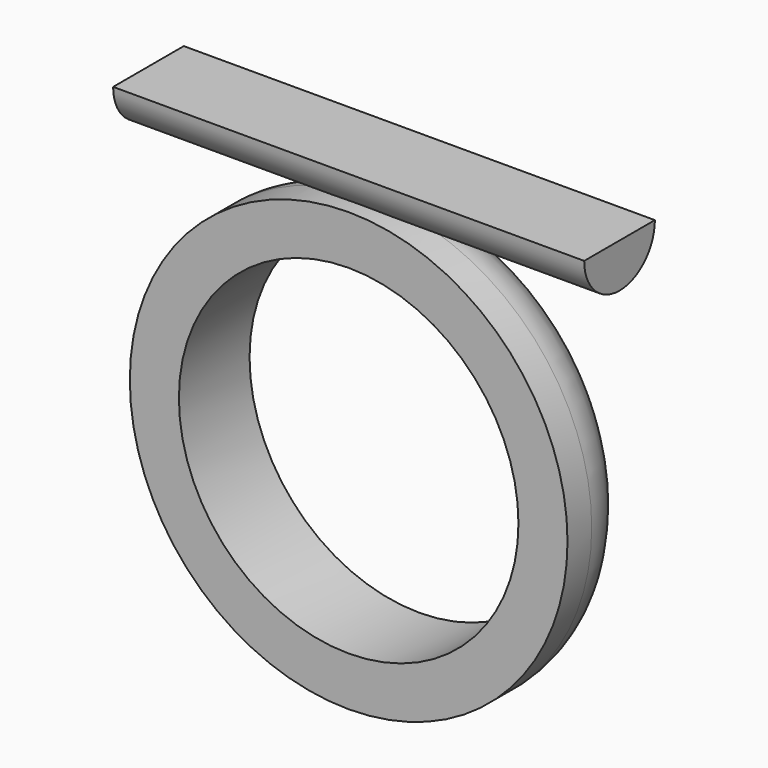
from build123d import *

# Parameters (mm, degrees)
F0_R          = 8.65
F1_DEPTH      = 2.25
F1_DEPTH_BACK = 2.25
F3_DEPTH      = 12
F3_DEPTH_BACK = 12
F4_S5_R       = 2.25
F4_T6_DEPTH   = 19


# Not quite as in the source:
# - a fillet or chamfer that OpenCascade refuses, or shapes differently, is made with other operations: its cross-section is extruded or revolved along the edge and cut away or added
# - a feature names something its author has since deleted; it is built from what else it names


with BuildPart() as f1:
    # F0 (on Front) → F1 (new body, two sides)
    with BuildSketch(Plane.XZ) as f1_sk:
        with BuildLine():
            ThreePointArc((-11.15, 0), (0, -11.15), (11.15, 0))
            ThreePointArc((11.15, 0), (7.8842406102, 7.8842406102), (0, 11.15))
            ThreePointArc((0, 11.15), (-7.8842406102, 7.8842406102), (-11.15, 0))
        make_face()
        Circle(F0_R, mode=Mode.SUBTRACT)
    extrude(amount=F1_DEPTH)
    extrude(f1_sk.sketch, amount=-F1_DEPTH_BACK)

    # F2 (on Right) → F3 (join, two sides)
    with BuildSketch(Plane.YZ) as f3_sk:
        with BuildLine():
            ThreePointArc((-2.25, 12.8644379824), (0, 10.6144379824), (2.25, 12.8644379824))
            Line((2.25, 12.8644379824), (0, 12.8644379824))
            Line((0, 12.8644379824), (-2.25, 12.8644379824))
        make_face()
    extrude(amount=F3_DEPTH)
    extrude(f3_sk.sketch, amount=-F3_DEPTH_BACK)

    # F4: fillet of radius 3 on 1 edges, made by hand


with BuildPart() as f4_tool2:
    # F4_s3 → F4_t4 (revolve)
    with BuildSketch(Plane.XY):
        with BuildLine():
            ThreePointArc((11.15, -0.7080398916), (10.4412878475, 1.2284517816), (8.65, 2.25))
            Line((8.65, 2.25), (11.15, 2.25))
            Line((11.15, 2.25), (11.15, -0.7080398916))
        make_face()
    revolve(axis=Axis((0, 2.25, 0), (0, -1, 0)))

    # F4_s5 → F4_t6 (cut, symmetric)
    with BuildSketch(Plane.YZ):
        with Locations((0, 12.8644379824)):
            Circle(F4_S5_R)
    extrude(amount=F4_T6_DEPTH, both=True, mode=Mode.SUBTRACT)


with BuildPart() as f1_1:
    add(f1.part)

    # F4_t1: cut F4_tool2
    add(f4_tool2.part, mode=Mode.SUBTRACT)


solid = f1_1.part
